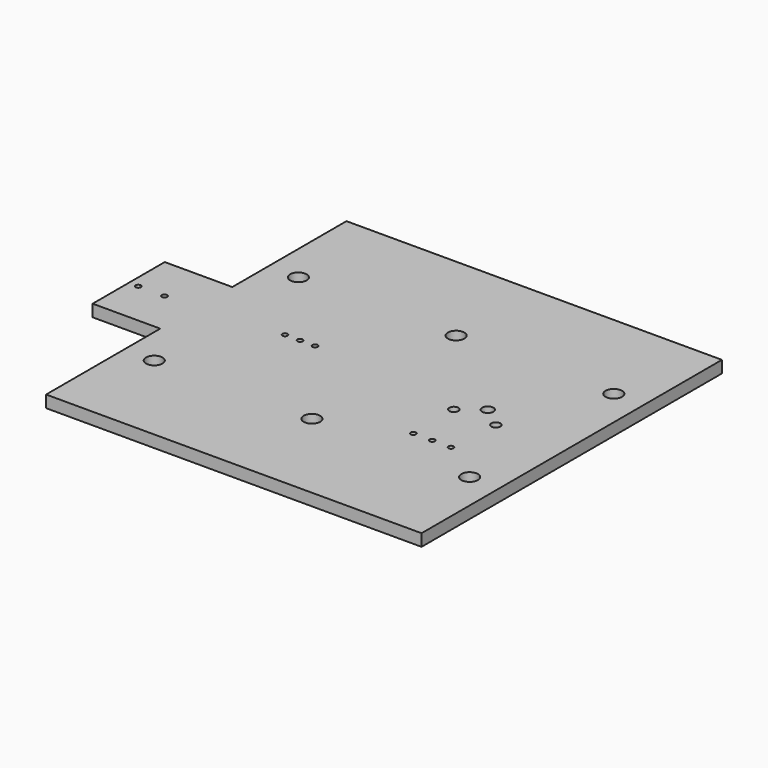
from build123d import *

# Parameters (mm, degrees)
F0_W     = 9
F0_H     = 12
F0_W_2   = 50
F0_H_2   = 19
F1_DEPTH = 1.6
F4_R     = 0.35
F5_R     = 0.35
F2_R     = 0.35
F6_DEPTH = 4
F7_R     = 1.1
F8_DEPTH = 25


# Not quite as in the source:
# - a feature names something its author has since deleted; it is built from what else it names


with BuildPart() as f1:
    # F0 (on Top) → F1 (new body)
    with BuildSketch(Plane.XY):
        with Locations((11.8172904253, 14.6750973295)):
            Rectangle(F0_W, F0_H)
        with Locations((41.3172904253, 14.6750973295)):
            Rectangle(F0_W_2, F0_H)
        with Locations((41.3172904253, -0.8249026705)):
            Rectangle(F0_W_2, F0_H_2)
        with Locations((41.3172904253, 30.1750973295)):
            Rectangle(F0_W_2, F0_H_2)
    extrude(amount=F1_DEPTH)

    # F4 (on face) + F5 (on face) + F3 (on face) + F2 (on face) → F6 (cut)
    with BuildSketch(Plane.XY.offset(1.6)):
        with Locations((51.6172904253, 6.6970097786)):
            Circle(F4_R)
        with Locations((56.6172904253, 6.6970097786)):
            Circle(F4_R)
        with Locations((54.1172904253, 6.6970097786)):
            Circle(F4_R)
    with BuildSketch(Plane.XY.offset(1.6)):
        with Locations((8.5672904253, 14.6970097786)):
            Circle(F5_R)
        with Locations((12.0672904253, 14.6970097786)):
            Circle(F5_R)
    with BuildSketch(Plane.XY.offset(1.6)):
        with BuildLine():
            Line((54.8172904253, 15.4470097786), (53.8172904253, 15.4470097786))
            ThreePointArc((53.8172904253, 15.4470097786), (53.640513733, 15.5202330803), (53.5672904253, 15.6970097701))
            ThreePointArc((53.5672904253, 15.6970097701), (54.3172904296, 14.9470097786), (55.0672904253, 15.6970097786))
            ThreePointArc((55.0672904253, 15.6970097786), (54.9940671206, 15.5202330833), (54.8172904253, 15.4470097786))
        make_face()
        with BuildLine():
            ThreePointArc((53.5672904253, 15.6970097701), (53.640513733, 15.5202330803), (53.8172904253, 15.4470097786))
            Line((53.8172904253, 15.4470097786), (54.8172904253, 15.4470097786))
            ThreePointArc((54.8172904253, 15.4470097786), (54.9940671206, 15.5202330833), (55.0672904253, 15.6970097786))
            ThreePointArc((55.0672904253, 15.6970097786), (54.9940671206, 15.8737864739), (54.8172904253, 15.9470097786))
            Line((54.8172904253, 15.9470097786), (53.8172904253, 15.9470097786))
            ThreePointArc((53.8172904253, 15.9470097786), (53.640513727, 15.8737864709), (53.5672904253, 15.6970097701))
        make_face()
        with BuildLine():
            ThreePointArc((55.0672904253, 15.6970097786), (54.317290421, 16.4470097786), (53.5672904253, 15.6970097701))
            ThreePointArc((53.5672904253, 15.6970097701), (53.640513727, 15.8737864709), (53.8172904253, 15.9470097786))
            Line((53.8172904253, 15.9470097786), (54.8172904253, 15.9470097786))
            ThreePointArc((54.8172904253, 15.9470097786), (54.9940671206, 15.8737864739), (55.0672904253, 15.6970097786))
        make_face()
        with BuildLine():
            Line((51.1672904253, 13.7970097786), (51.8672904253, 13.7970097786))
            ThreePointArc((51.8672904253, 13.7970097786), (52.0440671206, 13.7237864739), (52.1172904253, 13.5470097786))
            ThreePointArc((52.1172904253, 13.5470097786), (51.5172904253, 14.1470097786), (50.9172904253, 13.5470097786))
            ThreePointArc((50.9172904253, 13.5470097786), (50.99051373, 13.7237864739), (51.1672904253, 13.7970097786))
        make_face()
        with BuildLine():
            ThreePointArc((52.1172904253, 13.5470097786), (52.0440671206, 13.7237864739), (51.8672904253, 13.7970097786))
            Line((51.8672904253, 13.7970097786), (51.1672904253, 13.7970097786))
            ThreePointArc((51.1672904253, 13.7970097786), (50.99051373, 13.7237864739), (50.9172904253, 13.5470097786))
            ThreePointArc((50.9172904253, 13.5470097786), (50.99051373, 13.3702330833), (51.1672904253, 13.2970097786))
            Line((51.1672904253, 13.2970097786), (51.8672904253, 13.2970097786))
            ThreePointArc((51.8672904253, 13.2970097786), (52.0440671206, 13.3702330833), (52.1172904253, 13.5470097786))
        make_face()
        with BuildLine():
            ThreePointArc((50.9172904253, 13.5470097786), (51.5172904253, 12.9470097786), (52.1172904253, 13.5470097786))
            ThreePointArc((52.1172904253, 13.5470097786), (52.0440671206, 13.3702330833), (51.8672904253, 13.2970097786))
            Line((51.8672904253, 13.2970097786), (51.1672904253, 13.2970097786))
            ThreePointArc((51.1672904253, 13.2970097786), (50.99051373, 13.3702330833), (50.9172904253, 13.5470097786))
        make_face()
        with BuildLine():
            Line((56.7672904253, 13.2970097786), (57.4672904253, 13.2970097786))
            ThreePointArc((57.4672904253, 13.2970097786), (57.6440671206, 13.3702330833), (57.7172904253, 13.5470097786))
            ThreePointArc((57.7172904253, 13.5470097786), (57.6440671206, 13.7237864739), (57.4672904253, 13.7970097786))
            Line((57.4672904253, 13.7970097786), (56.7672904253, 13.7970097786))
            ThreePointArc((56.7672904253, 13.7970097786), (56.59051373, 13.7237864739), (56.5172904253, 13.5470097786))
            ThreePointArc((56.5172904253, 13.5470097786), (56.59051373, 13.3702330833), (56.7672904253, 13.2970097786))
        make_face()
        with BuildLine():
            ThreePointArc((57.7172904253, 13.5470097786), (57.6440671206, 13.3702330833), (57.4672904253, 13.2970097786))
            Line((57.4672904253, 13.2970097786), (56.7672904253, 13.2970097786))
            ThreePointArc((56.7672904253, 13.2970097786), (56.59051373, 13.3702330833), (56.5172904253, 13.5470097786))
            ThreePointArc((56.5172904253, 13.5470097786), (57.1172904253, 12.9470097786), (57.7172904253, 13.5470097786))
        make_face()
        with BuildLine():
            ThreePointArc((57.4672904253, 13.7970097786), (57.6440671206, 13.7237864739), (57.7172904253, 13.5470097786))
            ThreePointArc((57.7172904253, 13.5470097786), (57.1172904253, 14.1470097786), (56.5172904253, 13.5470097786))
            ThreePointArc((56.5172904253, 13.5470097786), (56.59051373, 13.7237864739), (56.7672904253, 13.7970097786))
            Line((56.7672904253, 13.7970097786), (57.4672904253, 13.7970097786))
        make_face()
    with BuildSketch(Plane.XY.offset(1.6)):
        with Locations((27.3172904253, 15.6970097786)):
            Circle(F2_R)
        with Locations((29.3172904253, 15.6970097786)):
            Circle(F2_R)
        with Locations((31.3172904253, 15.6970097786)):
            Circle(F2_R)
    extrude(amount=-F6_DEPTH, mode=Mode.SUBTRACT)

    # F7 (on face) → F8 (cut)
    with BuildSketch(Plane.XY.offset(1.6)):
        with Locations((62.3172904253, 26.6750973295)):
            Circle(F7_R)
        with Locations((20.3172904253, 26.6750973295)):
            Circle(F7_R)
        with Locations((62.3172904253, 2.6750973295)):
            Circle(F7_R)
        with Locations((20.3172904253, 2.6750973295)):
            Circle(F7_R)
        with Locations((41.3172904253, 2.6750973295)):
            Circle(F7_R)
        with Locations((41.3172904253, 26.6750973295)):
            Circle(F7_R)
    extrude(amount=-F8_DEPTH, mode=Mode.SUBTRACT)


solid = f1.part
